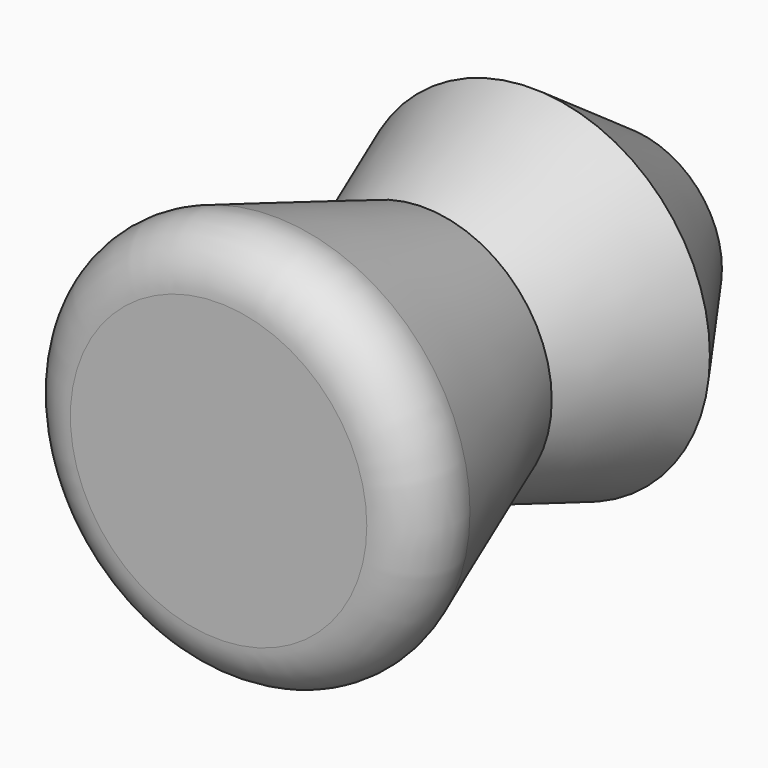
from build123d import *

# Parameters (mm, degrees)
F0_R     = 63.5
F1_DEPTH = 127
F1_TAPER = -20
F2_R     = 25.4
F3_SIZE  = 63.5


with BuildPart() as f1:
    # F0 (on Front) → F1 (new body, symmetric)
    with BuildSketch(Plane.XZ):
        Circle(F0_R)
    extrude(amount=F1_DEPTH, both=True, taper=F1_TAPER)

    # F2
    f2_edges = [f1.edges().sort_by_distance(p)[0] for p in [
        (-109.72422, -127, 0),
    ]]
    fillet(f2_edges, radius=F2_R)

    # F3
    f3_edges = [f1.edges().sort_by_distance(p)[0] for p in [
        (-109.72422, 127, 0),
    ]]
    chamfer(f3_edges, length=F3_SIZE)


solid = f1.part
